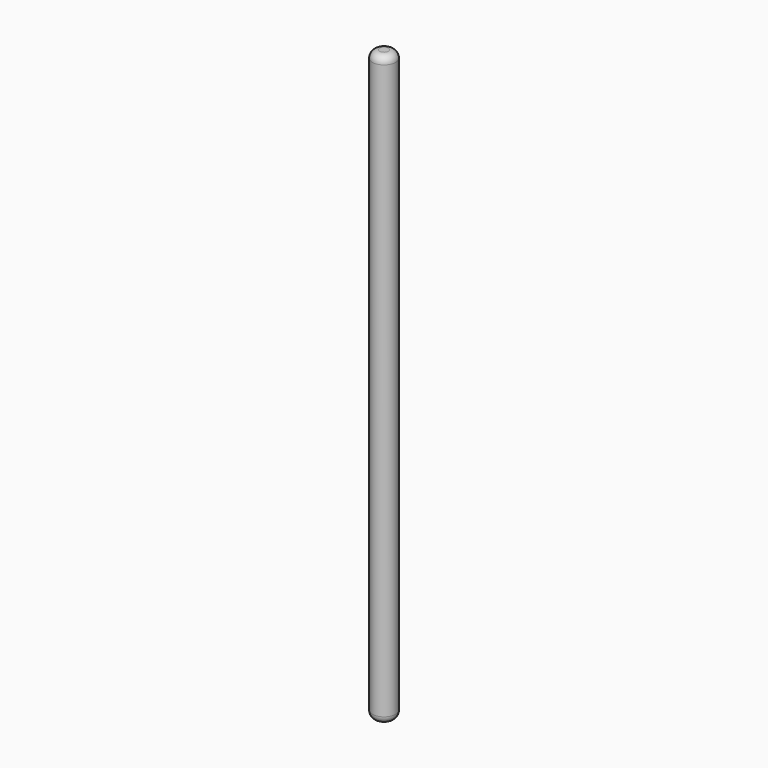
from build123d import *

# Parameters (mm, degrees)
F1_R     = 1.5875
F2_DEPTH = 80
F3_R     = 1


with BuildPart() as f2:
    # F1 (on Top) → F2 (new body)
    with BuildSketch(Plane.XY):
        Circle(F1_R)
    extrude(amount=F2_DEPTH)

    # F3
    f3_edges = [f2.edges().sort_by_distance(p)[0] for p in [
        (-1.5875, 0, 80),
        (-1.5875, 0, 0),
    ]]
    fillet(f3_edges, radius=F3_R)


solid = f2.part
